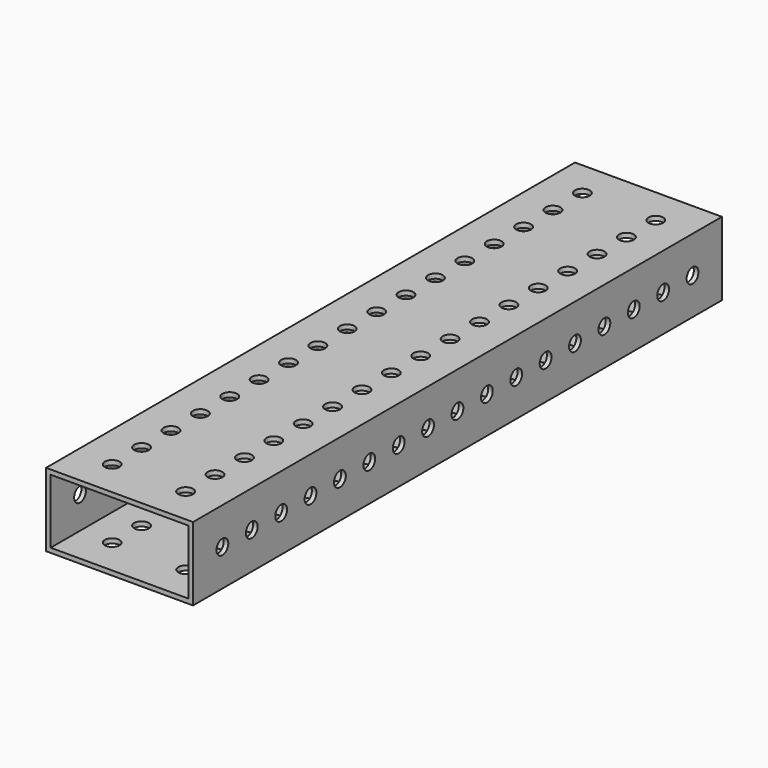
from build123d import *

# Parameters (mm, degrees)
F0_W     = 50.8
F0_H     = 25.4
F0_W_2   = 47.625
F0_H_2   = 22.225
F1_DEPTH = 228.6
F2_R     = 2.5527
F3_DEPTH = 279.4
F4_R     = 2.5527
F5_DEPTH = 25.4


# Not quite as in the source:
# - a feature names something its author has since deleted; it is built from what else it names


with BuildPart() as f1:
    # F0 (on Front) → F1 (new body)
    with BuildSketch(Plane.XZ):
        Rectangle(F0_W, F0_H)
        Rectangle(F0_W_2, F0_H_2, mode=Mode.SUBTRACT)
    extrude(amount=F1_DEPTH)

    # F2 (on face) → F3 (cut)
    with BuildSketch(Plane(origin=(-25.4, 0, 0), x_dir=(0, -1, 0), z_dir=(-1, 0, 0))):
        with Locations((12.7, 0)):
            Circle(F2_R)
        with Locations((25.4, 0)):
            Circle(F2_R)
        with Locations((38.1, 0)):
            Circle(F2_R)
        with Locations((50.8, 0)):
            Circle(F2_R)
        with Locations((63.5, 0)):
            Circle(F2_R)
        with Locations((88.9, 0)):
            Circle(F2_R)
        with Locations((101.6, 0)):
            Circle(F2_R)
        with Locations((76.2, 0)):
            Circle(F2_R)
        with Locations((114.3, 0)):
            Circle(F2_R)
        with Locations((127, 0)):
            Circle(F2_R)
        with Locations((139.7, 0)):
            Circle(F2_R)
        with Locations((152.4, 0)):
            Circle(F2_R)
        with Locations((165.1, 0)):
            Circle(F2_R)
        with Locations((177.8, 0)):
            Circle(F2_R)
        with Locations((190.5, 0)):
            Circle(F2_R)
        with Locations((203.2, 0)):
            Circle(F2_R)
        with Locations((215.9, 0)):
            Circle(F2_R)
    extrude(amount=-F3_DEPTH, mode=Mode.SUBTRACT)

    # F4 (on face) → F5 (cut)
    with BuildSketch(Plane(origin=(0, 0, -12.7), x_dir=(1, 0, 0), z_dir=(0, 0, -1))):
        with Locations((12.7, 25.4)):
            Circle(F4_R)
        with Locations((-12.7, 25.4)):
            Circle(F4_R)
        with Locations((-12.7, 127)):
            Circle(F4_R)
        with Locations((-12.7, 101.6)):
            Circle(F4_R)
        with Locations((12.7, 152.4)):
            Circle(F4_R)
        with Locations((-12.7, 177.8)):
            Circle(F4_R)
        with Locations((12.7, 63.5)):
            Circle(F4_R)
        with Locations((12.7, 190.5)):
            Circle(F4_R)
        with Locations((12.7, 101.6)):
            Circle(F4_R)
        with Locations((-12.7, 76.2)):
            Circle(F4_R)
        with Locations((-12.7, 139.7)):
            Circle(F4_R)
        with Locations((12.7, 12.7)):
            Circle(F4_R)
        with Locations((12.7, 76.2)):
            Circle(F4_R)
        with Locations((12.7, 50.8)):
            Circle(F4_R)
        with Locations((12.7, 88.9)):
            Circle(F4_R)
        with Locations((12.7, 139.7)):
            Circle(F4_R)
        with Locations((12.7, 177.8)):
            Circle(F4_R)
        with Locations((12.7, 165.1)):
            Circle(F4_R)
        with Locations((-12.7, 190.5)):
            Circle(F4_R)
        with Locations((12.7, 38.1)):
            Circle(F4_R)
        with Locations((-12.7, 38.1)):
            Circle(F4_R)
        with Locations((12.7, 203.2)):
            Circle(F4_R)
        with Locations((-12.7, 63.5)):
            Circle(F4_R)
        with Locations((12.7, 127)):
            Circle(F4_R)
        with Locations((-12.7, 165.1)):
            Circle(F4_R)
        with Locations((-12.7, 88.9)):
            Circle(F4_R)
        with Locations((12.7, 114.3)):
            Circle(F4_R)
        with Locations((-12.7, 114.3)):
            Circle(F4_R)
        with Locations((-12.7, 152.4)):
            Circle(F4_R)
        with Locations((-12.7, 203.2)):
            Circle(F4_R)
        with Locations((-12.7, 12.7)):
            Circle(F4_R)
        with Locations((-12.7, 50.8)):
            Circle(F4_R)
        with Locations((12.7, 215.9)):
            Circle(F4_R)
        with Locations((-12.7, 215.9)):
            Circle(F4_R)
    extrude(amount=-F5_DEPTH, mode=Mode.SUBTRACT)


solid = f1.part
